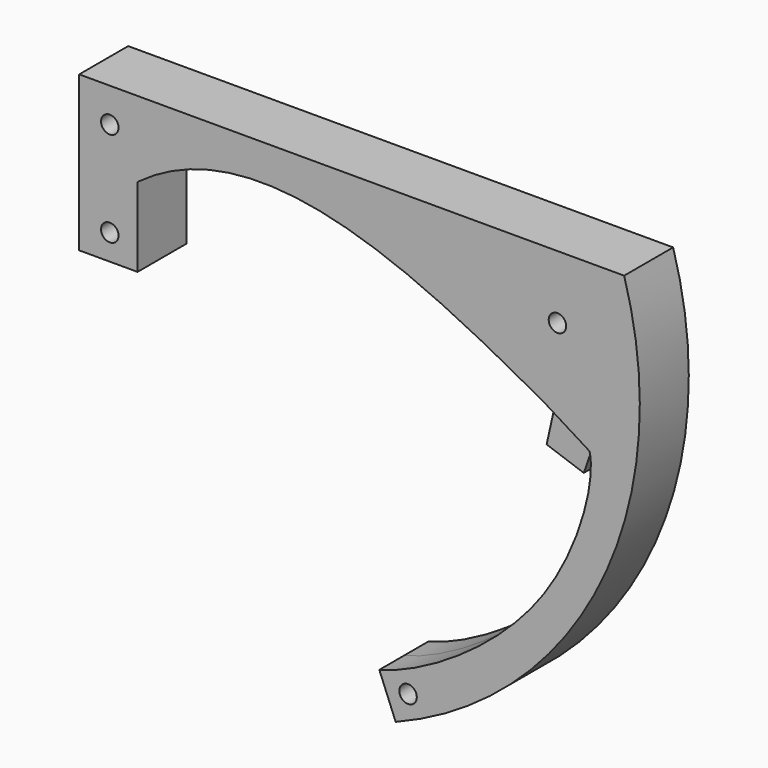
from build123d import *

# Parameters (mm, degrees)
F0_R     = 1
F1_DEPTH = 3.5
F2_DEPTH = 2.25


# Not quite as in the source:
# - a feature names something its author has since deleted; it is built from what else it names


with BuildPart() as f1:
    # F0 (on Front) → F1 (new body, symmetric)
    with BuildSketch(Plane.XZ):
        with BuildLine():
            Line((62.29, 21.44), (0, 21.44))
            Line((0, 21.44), (0, 3.7288318854))
            Line((0, 3.7288318854), (6.67, 3.7288318854))
            Line((6.67, 3.7288318854), (6.67, 12.7888318854))
            add(Edge.make_bspline(
                [(6.67, 12.7888318854), (20.3660801053, 23.045424372), (38.400747317, 13.8677307047), (52.300490874, 6.170732399)],
                knots=[0, 0, 0, 0, 46.1079270648, 46.1079270648, 46.1079270648, 46.1079270648], degree=3))
            Line((52.300490874, 6.170732399), (53.4860821652, 5.5017437759))
            Line((53.4860821652, 5.5017437759), (57.9021407774, 2.7602773683))
            Line((57.9021407774, 2.7602773683), (58.3288028571, 2.49540775))
            add(Edge.make_bspline(
                [(34.304166128, -27.3203667793), (39.4049563141, -26.0173317216), (55.1670315062, -16.4703750294), (59.0722335282, -0.2752133185), (58.3288028571, 2.49540775)],
                knots=[0, 0, 0, 0, 0.5353864124, 1, 1, 1, 1], degree=3))
            Line((34.304166128, -27.3203667793), (36.1752310606, -31.9570807038))
            ThreePointArc((36.1752310606, -31.9570807038), (59.6028549739, -10.3302859108), (62.29, 21.44))
        make_face()
        with Locations((37.5891347185, -28.6906498222)):
            Circle(F0_R, mode=Mode.SUBTRACT)
        with Locations((3.4974589944, 6.6614318639)):
            Circle(F0_R, mode=Mode.SUBTRACT)
        with Locations((3.4974589944, 17.5246726722)):
            Circle(F0_R, mode=Mode.SUBTRACT)
        with Locations((54.66741696, 14.1964312643)):
            Circle(F0_R, mode=Mode.SUBTRACT)
    extrude(amount=F1_DEPTH, both=True)

    # F0 (on Front) → F2 (join, symmetric)
    with BuildSketch(Plane.XZ):
        Polygon((56.6776084413, -0.7441981102), (57.9021407774, 2.7602773683), (53.4860821652, 5.5017437759), (52.4294775853, 0.7401819728), align=None)
    extrude(amount=F2_DEPTH, both=True)


solid = f1.part
